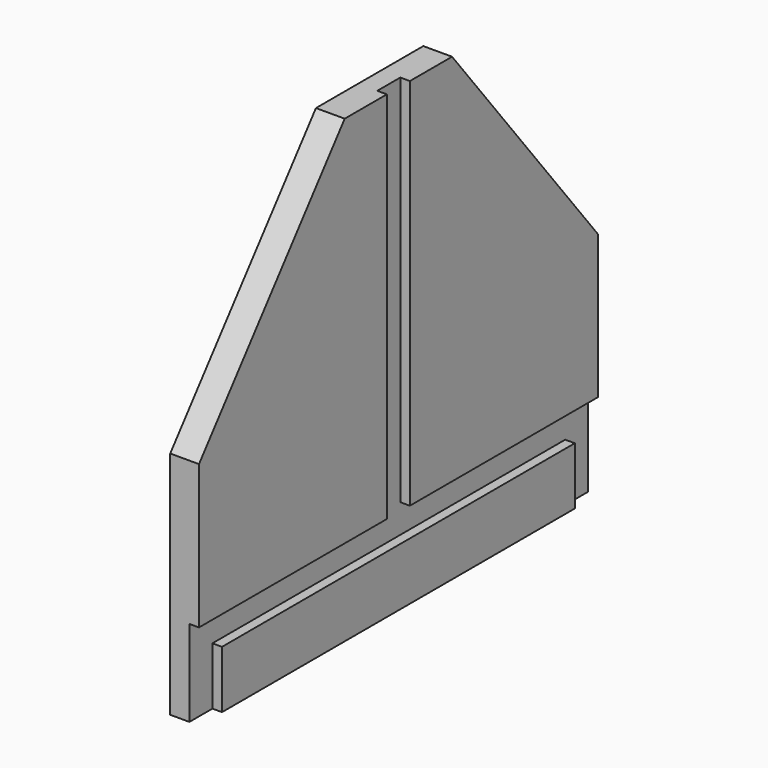
from build123d import *

# Parameters (mm, degrees)
F1_DEPTH = 19.05
F2_W     = 6.35
F2_H     = 19.05
F3_DEPTH = 330.2
F4_W     = 6.35
F4_H     = 19.05
F5_DEPTH = 38.1
F6_W     = 6.35
F6_H     = 19.05
F7_DEPTH = 247.65


# Not quite as in the source:
# - a feature names something its author has since deleted; it is built from what else it names


with BuildPart() as f1:
    # F0 (on Right) → F1 (new body)
    with BuildSketch(Plane.YZ):
        Polygon((-120.65, 27.2672971964), (-120.65, -125.1327028036), (209.55, -125.1327028036), (209.55, 27.2672971964), (88.9, 179.6672971964), (0, 179.6672971964), align=None)
    extrude(amount=F1_DEPTH)

    # F2 (on face) → F3 (cut)
    with BuildSketch(Plane.XZ.offset(120.65)):
        with Locations((15.875, -77.5077028036)):
            Rectangle(F2_W, F2_H)
    extrude(amount=-F3_DEPTH, mode=Mode.SUBTRACT)

    # F4 (on face) → F5 (cut)
    with BuildSketch(Plane(origin=(0, 0, -125.1327028036), x_dir=(1, 0, 0), z_dir=(0, 0, -1))):
        with Locations((15.875, 111.125)):
            Rectangle(F4_W, F4_H)
        with Locations((15.875, -200.025)):
            Rectangle(F4_W, F4_H)
    extrude(amount=-F5_DEPTH, mode=Mode.SUBTRACT)

    # F6 (on face) → F7 (cut)
    with BuildSketch(Plane.XY.offset(179.6672971964)):
        with Locations((15.875, 44.45)):
            Rectangle(F6_W, F6_H)
    extrude(amount=-F7_DEPTH, mode=Mode.SUBTRACT)


solid = f1.part
